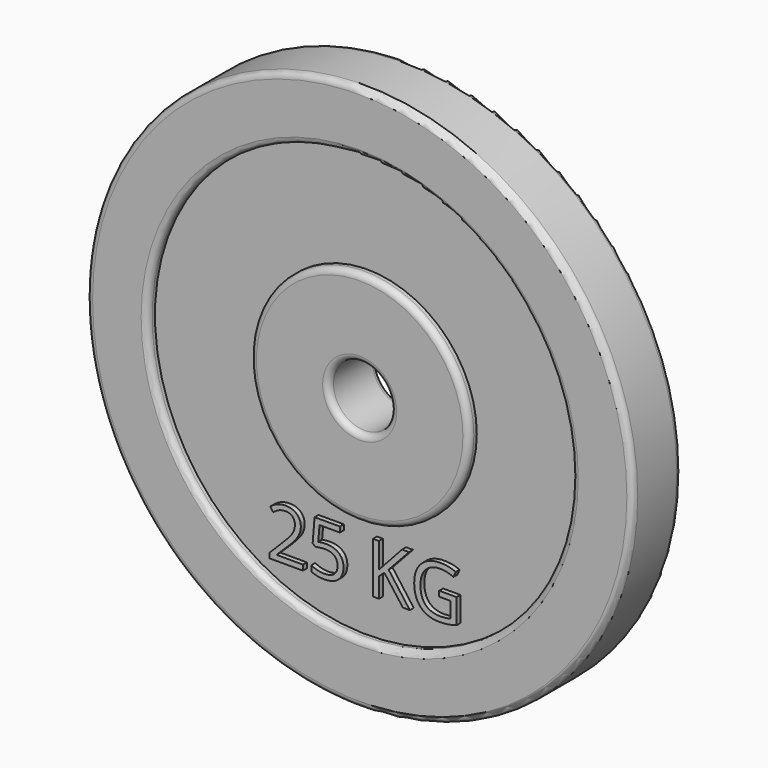
from build123d import *

# Parameters (mm, degrees)
F0_R         = 225
F0_R_2       = 25.5
F1_DEPTH     = 50
F2_R         = 5
F3_R         = 175
F3_R_2       = 90
F4_DEPTH     = 8
F5_R         = 175
F5_R_2       = 90
F6_DEPTH     = 8
F7_R         = 5
F8_TEXT_SIZE = 58.7192133107
F9_DEPTH     = 4


# Not quite as in the source:
# - Text() gives the source's letters only with a copy of the font that has no kerning and outlines rounded to 1/6400 em; it was checked with that copy


with BuildPart() as f1:
    # F0 (on Front) → F1 (new body)
    with BuildSketch(Plane.XZ):
        Circle(F0_R)
        Circle(F0_R_2, mode=Mode.SUBTRACT)
    extrude(amount=F1_DEPTH)

    # F2
    f2_edges = [f1.edges().sort_by_distance(p)[0] for p in [
        (-225, -50, 0),
        (-25.5, -50, 0),
        (-225, 0, 0),
        (-25.5, 0, 0),
    ]]
    fillet(f2_edges, radius=F2_R)

    # F3 (on face) → F4 (cut)
    with BuildSketch(Plane(origin=(0, 0, 0), x_dir=(-1, 0, 0), z_dir=(0, 1, 0))):
        Circle(F3_R)
        Circle(F3_R_2, mode=Mode.SUBTRACT)
    extrude(amount=-F4_DEPTH, mode=Mode.SUBTRACT)

    # F5 (on face) → F6 (cut)
    with BuildSketch(Plane.XZ.offset(50)):
        Circle(F5_R)
        Circle(F5_R_2, mode=Mode.SUBTRACT)
    extrude(amount=-F6_DEPTH, mode=Mode.SUBTRACT)

    # F7
    f7_edges = [f1.edges().sort_by_distance(p)[0] for p in [
        (-90, -50, 0),
        (-30.5, -50, 0),
        (-175, -50, 0),
        (175, 0, 0),
        (90, 0, 0),
    ]]
    fillet(f7_edges, radius=F7_R)


with BuildPart() as f9:
    # F8 (on face) → F9 (new body)
    with BuildSketch(Plane.XZ.offset(42)):
        with Locations((-80.3489860264, -143.013877931)):
            Text('25 KG', F8_TEXT_SIZE, font='Open Sans', text_align=(TextAlign.LEFT, TextAlign.BOTTOM))
    extrude(amount=F9_DEPTH)


solid = Compound([f1.part, f9.part])
